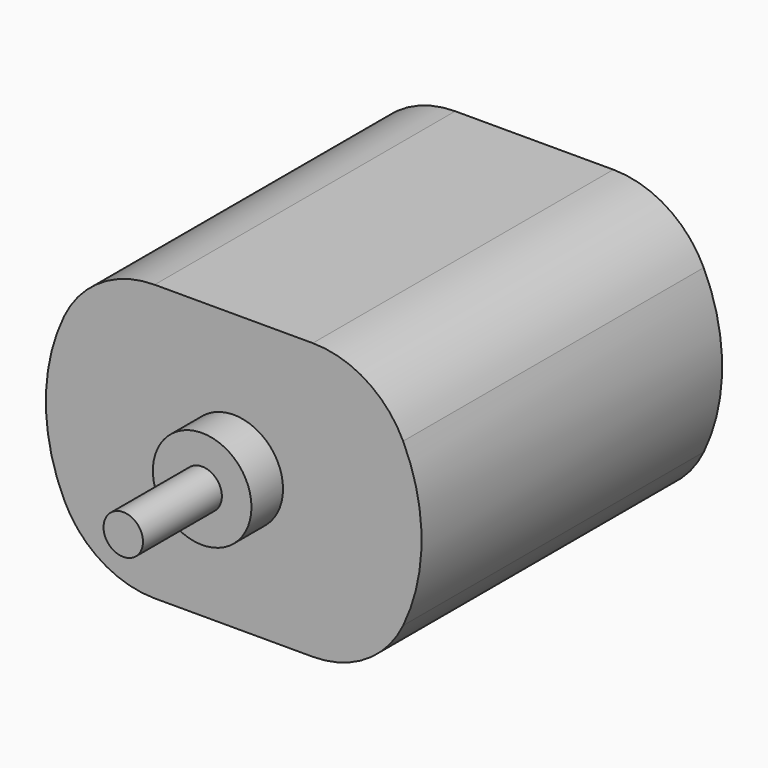
from build123d import *

# Parameters (mm, degrees)
F1_DEPTH  = 19.05
F2_R      = 5.08
F3_R      = 2.5
F4_DEPTH  = 2
F5_R      = 1
F6_DEPTH  = 5
F8_DEPTH  = 3.175
F9_R      = 1
F10_DEPTH = 1
F12_ANGLE = 90


# Not quite as in the source:
# - a length typed as a fraction of an inch, garbled in the dataset ("3 / 203.2 mm" for 3/8 in), is restored


with BuildPart() as f1:
    # F0 (on Top) → F1 (new body)
    with BuildSketch(Plane.XY):
        with BuildLine():
            Line((0, 7), (-6.4595375221, 7))
            ThreePointArc((-6.4595375221, 7), (-9.525, 0), (-6.4595375221, -7))
            Line((-6.4595375221, -7), (6.4595375221, -7))
            ThreePointArc((6.4595375221, -7), (9.525, 0), (6.4595375221, 7))
            Line((6.4595375221, 7), (0, 7))
        make_face()
    extrude(amount=F1_DEPTH)

    # F2
    f2_edges = [f1.edges().sort_by_distance(p)[0] for p in [
        (-6.459538, -7, 9.525),
        (6.459538, -7, 9.525),
        (-6.459538, 7, 9.525),
        (6.459538, 7, 9.525),
    ]]
    fillet(f2_edges, radius=F2_R)

    # F3 (on face) → F4 (join)
    with BuildSketch(Plane.XY.offset(19.05)):
        Circle(F3_R)
    extrude(amount=F4_DEPTH)

    # F5 (on face) → F6 (join)
    with BuildSketch(Plane.XY.offset(21.05)):
        Circle(F5_R)
    extrude(amount=F6_DEPTH)

    # F7 (on face) → F8 (join)
    with BuildSketch(Plane(origin=(0, 0, 0), x_dir=(1, 0, 0), z_dir=(0, 0, -1))):
        with BuildLine():
            Line((0, -3.5), (3.2297687611, -3.5))
            ThreePointArc((3.2297687611, -3.5), (0, 4.7625), (-3.2297687611, -3.5))
            Line((-3.2297687611, -3.5), (0, -3.5))
        make_face()
    extrude(amount=F8_DEPTH)

    # F9 (on face) → F10 (join)
    with BuildSketch(Plane(origin=(0, 0, -3.175), x_dir=(1, 0, 0), z_dir=(0, 0, -1))):
        Circle(F9_R)
    extrude(amount=F10_DEPTH)


with BuildPart() as f1_1:
    # F12: moved
    add(f1.part.rotate(Axis((1.8931087106, 0, 0), (1, 0, 0)), F12_ANGLE))


solid = f1_1.part
